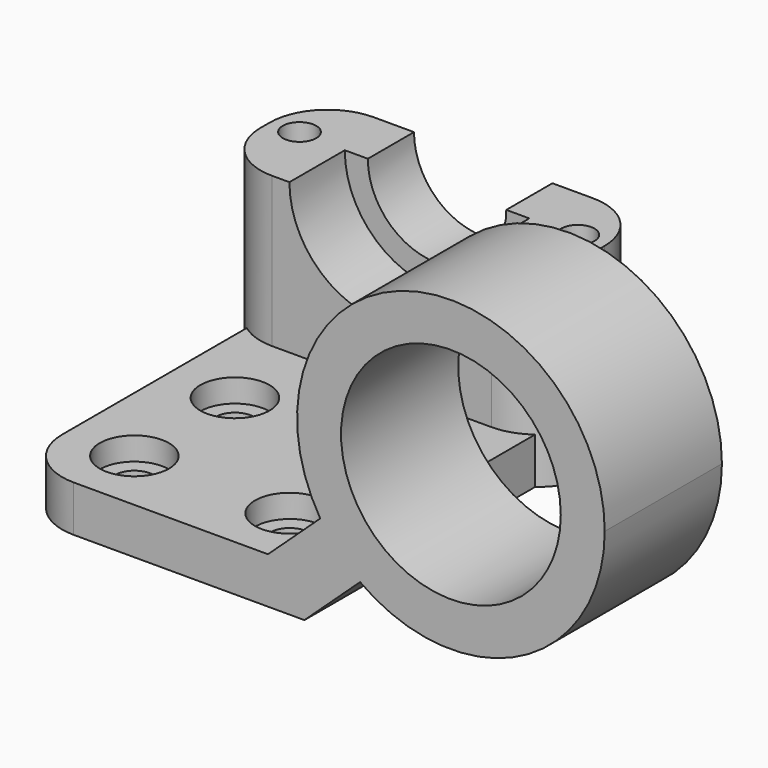
from build123d import *

# Parameters (mm, degrees)
F0_W      = 25
F0_H      = 35
F1_DEPTH  = 4
F2_R      = 1.675
F3_DEPTH  = 25
F4_W      = 25
F4_H      = 11
F5_DEPTH  = 13
F7_DEPTH  = 6
F8_R      = 8
F9_DEPTH  = 6
F2_R_2    = 3
F10_DEPTH = 2
F11_W     = 11
F11_H     = 17
F12_DEPTH = 2
F13_W     = 11
F13_H     = 17
F14_DEPTH = 2
F15_R     = 1.45
F16_DEPTH = 25
F17_R     = 5
F18_R     = 9.525
F19_DEPTH = 12.7
F20_R     = 5


with BuildPart() as f1:
    # F0 (on Top) → F1 (new body)
    with BuildSketch(Plane.XY):
        with Locations((12.5, 17.5)):
            Rectangle(F0_W, F0_H)
    extrude(amount=F1_DEPTH)

    # F2 (on face) → F3 (cut)
    with BuildSketch(Plane.XY.offset(4)):
        with BuildLine():
            ThreePointArc((4.094, 16.5088346784), (5.769, 14.8338346784), (7.444, 16.5088346784))
            ThreePointArc((7.444, 16.5088346784), (5.769, 18.1838346784), (4.094, 16.5088346784))
        make_face()
        with Locations((19.231, 16.5088346784)):
            Circle(F2_R)
        with Locations((19.231, 5.6122346784)):
            Circle(F2_R)
        with Locations((5.769, 5.6122346784)):
            Circle(F2_R)
    extrude(amount=-F3_DEPTH, mode=Mode.SUBTRACT)

    # F4 (on face) → F5 (join)
    with BuildSketch(Plane.XY.offset(4)):
        with Locations((12.5, 29.5)):
            Rectangle(F4_W, F4_H)
    extrude(amount=F5_DEPTH)

    # F6 (on face) → F7 (cut)
    with BuildSketch(Plane(origin=(0, 35, 0), x_dir=(-1, 0, 0), z_dir=(0, 1, 0))):
        with BuildLine():
            ThreePointArc((-18.5, 17), (-12.5, 11), (-6.5, 17))
            Line((-6.5, 17), (-18.5, 17))
        make_face()
    extrude(amount=-F7_DEPTH, mode=Mode.SUBTRACT)

    # F8 (on face) → F9 (cut)
    with BuildSketch(Plane.XZ.offset(-24)):
        with Locations((12.5, 17)):
            Circle(F8_R)
    extrude(amount=-F9_DEPTH, mode=Mode.SUBTRACT)

    # F2 (on face) → F10 (cut)
    with BuildSketch(Plane.XY.offset(4)):
        with BuildLine():
            ThreePointArc((8.769, 16.5088346784), (5.769, 19.5088346784), (2.769, 16.5088346784))
            ThreePointArc((2.769, 16.5088346784), (5.769, 13.5088346784), (8.769, 16.5088346784))
        make_face()
        with BuildLine():
            ThreePointArc((4.094, 16.5088346784), (5.769, 18.1838346784), (7.444, 16.5088346784))
            ThreePointArc((7.444, 16.5088346784), (5.769, 14.8338346784), (4.094, 16.5088346784))
        make_face(mode=Mode.SUBTRACT)
        with Locations((19.231, 16.5088346784)):
            Circle(F2_R_2)
        with Locations((19.231, 16.5088346784)):
            Circle(F2_R, mode=Mode.SUBTRACT)
        with Locations((19.231, 5.6122346784)):
            Circle(F2_R_2)
        with Locations((19.231, 5.6122346784)):
            Circle(F2_R, mode=Mode.SUBTRACT)
        with Locations((5.769, 5.6122346784)):
            Circle(F2_R_2)
        with Locations((5.769, 5.6122346784)):
            Circle(F2_R, mode=Mode.SUBTRACT)
    extrude(amount=-F10_DEPTH, mode=Mode.SUBTRACT)

    # F11 (on face) → F12 (join)
    with BuildSketch(Plane(origin=(0, 0, 0), x_dir=(0, -1, 0), z_dir=(-1, 0, 0))):
        with Locations((-29.5, 8.5)):
            Rectangle(F11_W, F11_H)
    extrude(amount=F12_DEPTH)

    # F13 (on face) → F14 (join)
    with BuildSketch(Plane.YZ.offset(25)):
        with Locations((29.5, 8.5)):
            Rectangle(F13_W, F13_H)
    extrude(amount=F14_DEPTH)

    # F15 (on face) → F16 (cut)
    with BuildSketch(Plane.XY.offset(17)):
        with Locations((0.4384, 30.174)):
            Circle(F15_R)
        with Locations((24.5616, 30.174)):
            Circle(F15_R)
    extrude(amount=-F16_DEPTH, mode=Mode.SUBTRACT)

    # F17
    f17_edges = [f1.edges().sort_by_distance(p)[0] for p in [
        (-2, 24, 8.5),
        (-2, 35, 8.5),
        (27, 35, 8.5),
        (27, 24, 8.5),
    ]]
    fillet(f17_edges, radius=F17_R)

    # F18 (on face) → F19 (join)
    with BuildSketch(Plane.XZ):
        with BuildLine():
            Line((26.3737617011, 8.2016371934), (29.8278119435, 4.4765953247))
            ThreePointArc((29.8278119435, 4.4765953247), (43.7351717982, 3.3488719473), (51.035, 15.24))
            ThreePointArc((51.035, 15.24), (34.0402980118, 28.0629796209), (26.3737617011, 8.2016371934))
        make_face()
        with Locations((37.7, 15.24)):
            Circle(F18_R, mode=Mode.SUBTRACT)
        with BuildLine():
            Line((25, 4), (25, 0))
            Line((25, 0), (29.8278119435, 4.4765953247))
            ThreePointArc((29.8278119435, 4.4765953247), (27.9217650948, 6.1731181138), (26.3737617011, 8.2016371934))
            Line((26.3737617011, 8.2016371934), (21.8424800567, 4))
            Line((21.8424800567, 4), (25, 4))
        make_face()
        with BuildLine():
            ThreePointArc((26.3737617011, 8.2016371934), (27.9217650948, 6.1731181138), (29.8278119435, 4.4765953247))
            Line((29.8278119435, 4.4765953247), (26.3737617011, 8.2016371934))
        make_face()
    extrude(amount=-F19_DEPTH)

    # F20
    f20_edges = [f1.edges().sort_by_distance(p)[0] for p in [
        (0, 0, 2),
    ]]
    fillet(f20_edges, radius=F20_R)


solid = f1.part
